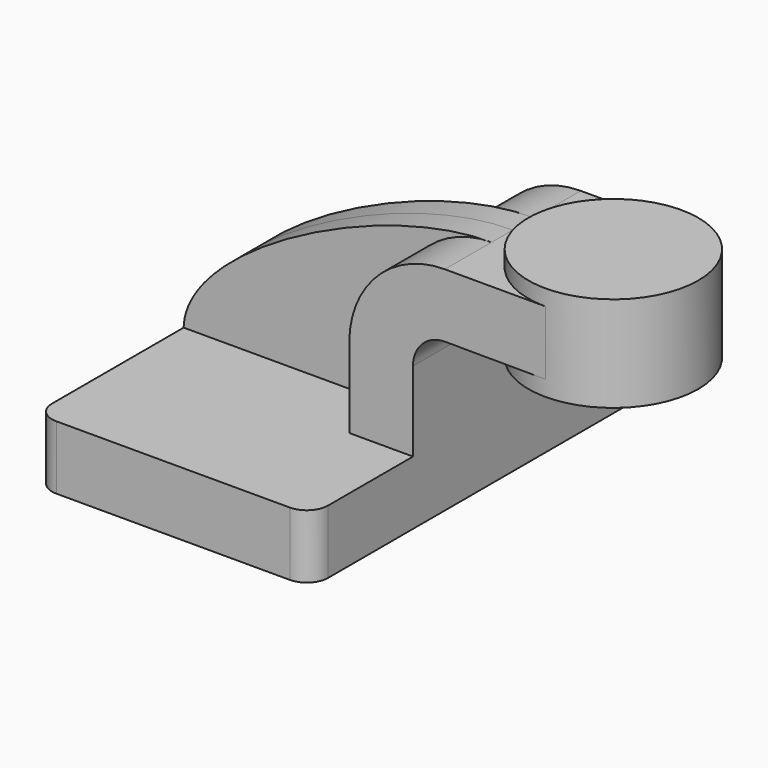
from build123d import *

# Parameters (mm, degrees)
F1_DEPTH = 63.5
F2_DEPTH = 25.4
F3_DEPTH = 7.9375
F5_R     = 6.35


with BuildPart() as f1:
    # F0 (on Front) → F1 (new body, symmetric)
    with BuildSketch(Plane.XZ):
        Polygon((-41.275, -9.525), (41.275, -9.525), (41.275, 9.525), (22.225, 9.525), (-41.275, 9.525), align=None)
    extrude(amount=F1_DEPTH, both=True)

    # F0 (on Front) → F2 (join, symmetric)
    with BuildSketch(Plane.XZ):
        with BuildLine():
            Line((22.225, 9.525), (41.275, 9.525))
            Line((41.275, 9.525), (41.275, 33.3553104297))
            ThreePointArc((41.275, 33.3553104297), (44.063311099, 40.086888901), (50.7948895703, 42.8752))
            Line((50.7948895703, 42.8752), (55.4659834841, 42.8752))
            Line((55.4659834841, 42.8752), (55.4659834841, 61.9252))
            Line((55.4659834841, 61.9252), (50.7948895703, 61.9252))
            ThreePointArc((50.7948895703, 61.9252), (30.5929269174, 53.5572730826), (22.225, 33.3553104297))
            Line((22.225, 33.3553104297), (22.225, 9.525))
        make_face()
        Polygon((70.8683976346, 61.9252), (55.4659834841, 61.9252), (55.4659834841, 42.8752), (55.4659834841, 42.8555016406), (80.8659834841, 42.748387903), (80.8659834841, 61.9252), align=None)
    extrude(amount=F2_DEPTH, both=True)

    # F0 (on Front) → F3 (join, symmetric)
    with BuildSketch(Plane.XZ):
        with BuildLine():
            add(Edge.make_bspline(
                [(-41.275, 9.525), (-40.730714798, 32.5702540576), (17.2467883676, 62.170214951), (50.7948895703, 61.9252)],
                knots=[0, 0, 0, 0, 105.9369884673, 105.9369884673, 105.9369884673, 105.9369884673], degree=3))
            Line((-41.275, 9.525), (22.225, 9.525))
            Line((22.225, 9.525), (22.225, 33.3553104297))
            ThreePointArc((22.225, 33.3553104297), (30.5929269174, 53.5572730826), (50.7948895703, 61.9252))
        make_face()
    extrude(amount=F3_DEPTH, both=True)

    # F0 (on Front) → F4 (revolve)
    with BuildSketch(Plane.XZ):
        Polygon((80.8659834841, 61.9252), (80.8659834841, 42.748387903), (80.8659834841, 38.1), (106.2659834841, 38.1), (106.2659834841, 66.675), (80.8659834841, 66.675), align=None)
    revolve(axis=Axis((80.8659834841, 0, 52.3875), (0, 0, -1)))

    # F5
    f5_edges = [f1.edges().sort_by_distance(p)[0] for p in [
        (-41.275, -63.5, 0),
        (41.275, -63.5, 0),
        (41.275, 63.5, 0),
        (-41.275, 63.5, 0),
    ]]
    fillet(f5_edges, radius=F5_R)


solid = f1.part
